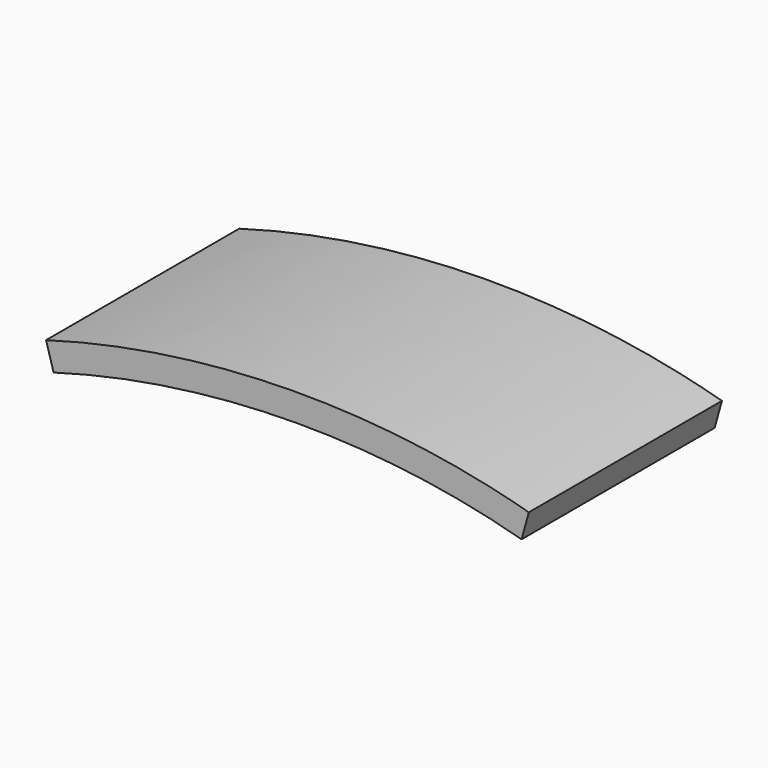
from build123d import *

# Parameters (mm, degrees)
F1_DEPTH = 1016


with BuildPart() as f1:
    # F0 (on Front) → F1 (new body)
    with BuildSketch(Plane.XZ):
        with BuildLine():
            add(Edge.make_bspline(
                [(-948.8851096128, 0), (-296.5447090113, 188.3144754409), (431.0441784436, 203.5579582314), (1083.1148903872, 22.7177995874)],
                knots=[0, 0, 0, 0, 2032.1269887529, 2032.1269887529, 2032.1269887529, 2032.1269887529], degree=3))
            Line((-948.8851096128, 0), (-917.1839899029, -109.8158868704))
            add(Edge.make_bspline(
                [(-917.1839899029, -109.8158868704), (-838.1638847431, -87.0047446528), (-677.7437282731, -46.595139966), (-431.7880751926, -1.941782143), (-182.328163559, 26.4501167169), (68.812065297, 38.3021262725), (319.8091103509, 33.3575818517), (568.8434154703, 11.3817690533), (814.1037690507, -27.8377449472), (973.896630374, -65.6066346054), (1052.5687682639, -87.4249460803)],
                knots=[0, 0, 0, 0, 0.125, 0.25, 0.375, 0.5, 0.625, 0.75, 0.875, 1, 1, 1, 1], degree=3))
            Line((1052.5687682639, -87.4249460803), (1083.1148903872, 22.7177995874))
        make_face()
    extrude(amount=F1_DEPTH)


solid = f1.part
